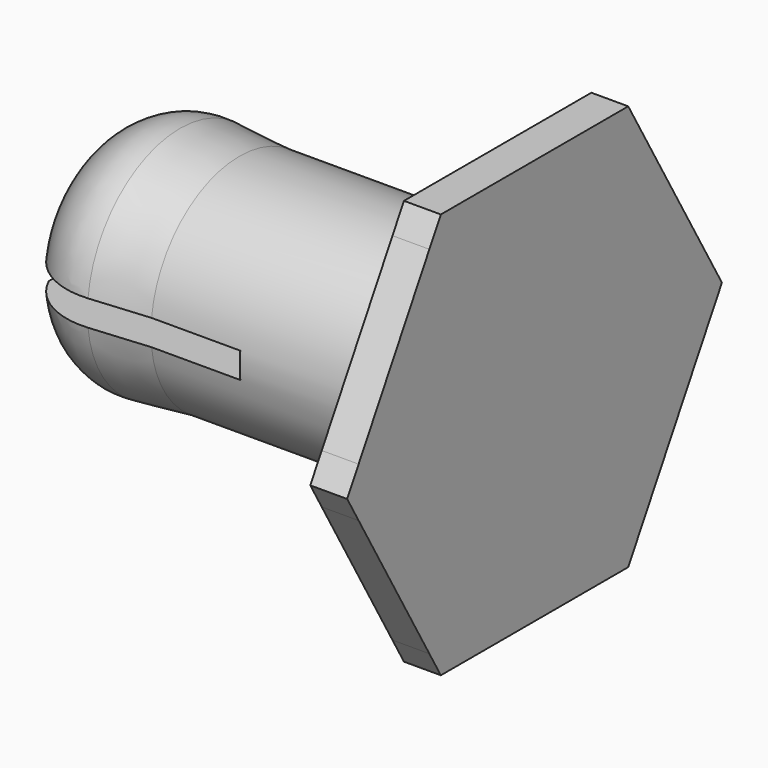
from build123d import *
from build123d import SkipClean  # not in build123d's __all__

# Parameters (mm, degrees)
F3_DEPTH = 6
F4_W     = 13.7017059222
F4_H     = 13
F4_R     = 3
F5_DEPTH = 25
F6_DEPTH = 1


with BuildPart() as f1:
    # F0 (on Front) → F1 (revolve)
    with BuildSketch(Plane.XZ):
        with BuildLine():
            Line((-11.5940445242, 0), (0, 0))
            Line((0, 0), (0, 6))
            Line((0, 6), (-1, 6))
            Line((-1, 6), (-1, 3))
            Line((-1, 3), (-8, 3))
            Line((-8, 3), (-9.6100640914, 3.1408623555))
            ThreePointArc((-9.6100640914, 3.1408623555), (-10.7813661664, 2.8822577685), (-11.5940445242, 2))
            Line((-11.5940445242, 2), (-11.5940445242, 0))
        make_face()
    revolve(axis=Axis((-5.7970222621, 0, 0), (1, 0, 0)))

    # F2 (on face) → F3 (cut)
    with BuildSketch(Plane(origin=(-11.5940445242, 0, 0), x_dir=(0, -1, 0), z_dir=(-1, 0, 0))):
        with BuildLine():
            ThreePointArc((-1.9691368668, -0.35), (-2, 0), (-1.9691368668, 0.35))
            Line((-1.9691368668, 0.35), (-4, 0.35))
            Line((-4, 0.35), (-4, -0.35))
            Line((-4, -0.35), (-2.9795133831, -0.35))
            Line((-2.9795133831, -0.35), (-1.9691368668, -0.35))
        make_face()
        with BuildLine():
            Line((1.9691368668, 0.35), (0.25, 0.35))
            Line((0.25, 0.35), (0.25, 0))
            Line((0.25, 0), (0.25, -0.35))
            Line((0.25, -0.35), (1.9691368668, -0.35))
            ThreePointArc((1.9691368668, -0.35), (1.9922692757, -0.1756790632), (2, 0))
            ThreePointArc((2, 0), (1.9922692757, 0.1756790632), (1.9691368668, 0.35))
        make_face()
        with BuildLine():
            Line((-0.25, 0), (-0.25, 0.35))
            Line((-0.25, 0.35), (-1.9691368668, 0.35))
            ThreePointArc((-1.9691368668, 0.35), (-2, 0), (-1.9691368668, -0.35))
            Line((-1.9691368668, -0.35), (-0.25, -0.35))
            Line((-0.25, -0.35), (-0.25, 0))
        make_face()
        Polygon((0.25, 0), (0.25, 0.35), (-0.25, 0.35), (-0.25, 0), (-0.25, -0.35), (0.25, -0.35), align=None)
        with BuildLine():
            Line((4, 0.35), (1.9691368668, 0.35))
            ThreePointArc((1.9691368668, 0.35), (1.9922692757, 0.1756790632), (2, 0))
            ThreePointArc((2, 0), (1.9922692757, -0.1756790632), (1.9691368668, -0.35))
            Line((1.9691368668, -0.35), (2.9795133831, -0.35))
            Line((2.9795133831, -0.35), (4, -0.35))
            Line((4, -0.35), (4, 0.35))
        make_face()
    extrude(amount=-F3_DEPTH, mode=Mode.SUBTRACT)

    # F4 (on face) → F5 (cut)
    with BuildSketch(Plane(origin=(-1, 0, 0), x_dir=(0, -1, 0), z_dir=(-1, 0, 0))):
        Rectangle(F4_W, F4_H)
        Polygon((-6.3508529611, 0), (-3.1754264805, 5.5), (3.1754264805, 5.5), (6.3508529611, 0), (3.1754264805, -5.5), (-3.1754264805, -5.5), align=None, mode=Mode.SUBTRACT)
        with BuildLine():
            Line((2.3979157617, 5.5), (-2.3979157617, 5.5))
            ThreePointArc((-2.3979157617, 5.5), (-3, 5.1961524227), (-3.56418184, 4.8266559657))
            Line((-3.56418184, 4.8266559657), (-5.9620976016, 0.6733440343))
            ThreePointArc((-5.9620976016, 0.6733440343), (-6, 0), (-5.9620976016, -0.6733440343))
            Line((-5.9620976016, -0.6733440343), (-3.56418184, -4.8266559657))
            ThreePointArc((-3.56418184, -4.8266559657), (-3, -5.1961524227), (-2.3979157617, -5.5))
            Line((-2.3979157617, -5.5), (2.3979157617, -5.5))
            ThreePointArc((2.3979157617, -5.5), (3, -5.1961524227), (3.56418184, -4.8266559657))
            Line((3.56418184, -4.8266559657), (5.9620976016, -0.6733440343))
            ThreePointArc((5.9620976016, -0.6733440343), (5.9905169063, -0.3372049749), (6, 0))
            ThreePointArc((6, 0), (5.9905169063, 0.3372049749), (5.9620976016, 0.6733440343))
            Line((5.9620976016, 0.6733440343), (3.56418184, 4.8266559657))
            ThreePointArc((3.56418184, 4.8266559657), (3, 5.1961524227), (2.3979157617, 5.5))
        make_face()
        Circle(F4_R, mode=Mode.SUBTRACT)
    with SkipClean():  # cleaning this boolean's faces spoils the solid; the shape is the same uncleaned
        extrude(amount=-F5_DEPTH, mode=Mode.SUBTRACT)

    # F4 (on face) → F6 (join)
    with BuildSketch(Plane(origin=(-1, 0, 0), x_dir=(0, -1, 0), z_dir=(-1, 0, 0))):
        with BuildLine():
            Line((2.3979157617, 5.5), (-2.3979157617, 5.5))
            ThreePointArc((-2.3979157617, 5.5), (-3, 5.1961524227), (-3.56418184, 4.8266559657))
            Line((-3.56418184, 4.8266559657), (-5.9620976016, 0.6733440343))
            ThreePointArc((-5.9620976016, 0.6733440343), (-6, 0), (-5.9620976016, -0.6733440343))
            Line((-5.9620976016, -0.6733440343), (-3.56418184, -4.8266559657))
            ThreePointArc((-3.56418184, -4.8266559657), (-3, -5.1961524227), (-2.3979157617, -5.5))
            Line((-2.3979157617, -5.5), (2.3979157617, -5.5))
            ThreePointArc((2.3979157617, -5.5), (3, -5.1961524227), (3.56418184, -4.8266559657))
            Line((3.56418184, -4.8266559657), (5.9620976016, -0.6733440343))
            ThreePointArc((5.9620976016, -0.6733440343), (5.9905169063, -0.3372049749), (6, 0))
            ThreePointArc((6, 0), (5.9905169063, 0.3372049749), (5.9620976016, 0.6733440343))
            Line((5.9620976016, 0.6733440343), (3.56418184, 4.8266559657))
            ThreePointArc((3.56418184, 4.8266559657), (3, 5.1961524227), (2.3979157617, 5.5))
        make_face()
        Circle(F4_R, mode=Mode.SUBTRACT)
        with BuildLine():
            Line((-2.3979157617, 5.5), (-3.1754264805, 5.5))
            Line((-3.1754264805, 5.5), (-3.56418184, 4.8266559657))
            ThreePointArc((-3.56418184, 4.8266559657), (-3, 5.1961524227), (-2.3979157617, 5.5))
        make_face()
        with BuildLine():
            Line((3.1754264805, 5.5), (2.3979157617, 5.5))
            ThreePointArc((2.3979157617, 5.5), (3, 5.1961524227), (3.56418184, 4.8266559657))
            Line((3.56418184, 4.8266559657), (3.1754264805, 5.5))
        make_face()
        with BuildLine():
            Line((6.3508529611, 0), (5.9620976016, 0.6733440343))
            ThreePointArc((5.9620976016, 0.6733440343), (5.9905169063, 0.3372049749), (6, 0))
            ThreePointArc((6, 0), (5.9905169063, -0.3372049749), (5.9620976016, -0.6733440343))
            Line((5.9620976016, -0.6733440343), (6.3508529611, 0))
        make_face()
        with BuildLine():
            ThreePointArc((3.56418184, -4.8266559657), (3, -5.1961524227), (2.3979157617, -5.5))
            Line((2.3979157617, -5.5), (3.1754264805, -5.5))
            Line((3.1754264805, -5.5), (3.56418184, -4.8266559657))
        make_face()
        with BuildLine():
            ThreePointArc((-2.3979157617, -5.5), (-3, -5.1961524227), (-3.56418184, -4.8266559657))
            Line((-3.56418184, -4.8266559657), (-3.1754264805, -5.5))
            Line((-3.1754264805, -5.5), (-2.3979157617, -5.5))
        make_face()
        with BuildLine():
            ThreePointArc((-5.9620976016, -0.6733440343), (-6, 0), (-5.9620976016, 0.6733440343))
            Line((-5.9620976016, 0.6733440343), (-6.3508529611, 0))
            Line((-6.3508529611, 0), (-5.9620976016, -0.6733440343))
        make_face()
    extrude(amount=-F6_DEPTH)


solid = f1.part
